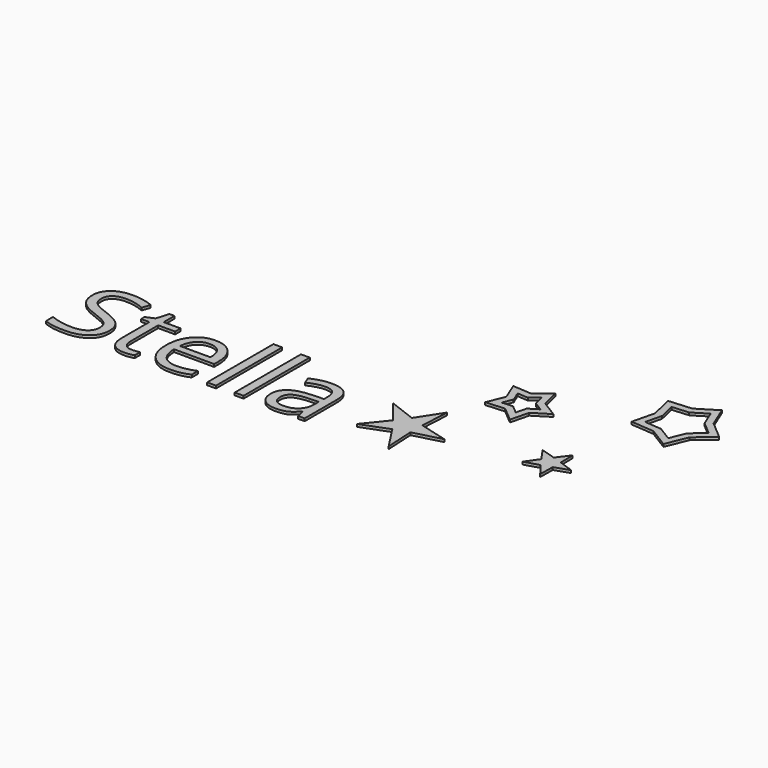
from build123d import *

# Parameters (mm, degrees)
F0_TEXT_SIZE = 12.7545618733
F1_DEPTH     = 0.3


# Not quite as in the source:
# - Text() gives the source's letters only with a copy of the font that has no kerning and outlines rounded to 1/6400 em; it was checked with that copy


with BuildPart() as f1:
    # F0 (on Top) → F1 (new body)
    with BuildSketch(Plane.XY):
        Polygon((45.5197678753, 19.2148680571), (42.8062423837, 19.0067321436), (43.4468188584, 16.3616985083), (42.8062423837, 13.7166648729), (45.5197678753, 13.5085289594), (47.8373953331, 12.0819441849), (48.8738698415, 14.5983427514), (50.9468188584, 16.3616985083), (48.8738698415, 18.1250542651), (47.8373953331, 20.6414528316), align=None)
        Polygon((47.4558552841, 19.467193304), (48.2079466306, 17.641232732), (49.7121293236, 16.3616985083), (48.2079466306, 15.0821642845), (47.4558552841, 13.2562037126), (45.7741279079, 14.2913686445), (43.8051272001, 14.4423971726), (44.2699452149, 16.3616985083), (43.8051272001, 18.2809998439), (45.7741279079, 18.4320283721), align=None, mode=Mode.SUBTRACT)
        Polygon((32.15595247, 12.3196945685), (29.9424269785, 12.4748299189), (30.7739864588, 10.4175815359), (29.9424269785, 8.3603331529), (32.15595247, 8.5154685033), (33.8555459391, 7.0888837288), (34.3920204475, 9.2420110313), (36.2739864588, 10.4175815359), (34.3920204475, 11.5931520405), (33.8555459391, 13.7462793429), align=None)
        Polygon((33.3889164299, 12.3101413844), (33.6939336388, 11.0859622857), (34.7639416466, 10.4175815359), (33.6939336388, 9.7492007861), (33.3889164299, 8.5250216874), (32.4225979039, 9.3361187653), (31.1640788938, 9.2479152238), (31.6368692086, 10.4175815359), (31.1640788938, 11.587247848), (32.4225979039, 11.4990443064), align=None, mode=Mode.SUBTRACT)
        Polygon((41.6785921238, 3.7183704865), (39.9650666323, 4.236777101), (40.9876091182, 2.7673139703), (39.9650666323, 1.2978508395), (41.6785921238, 1.816257454), (42.7601516042, 0.3896726795), (42.7966261126, 2.179528718), (44.4876091182, 2.7673139703), (42.7966261126, 3.3550992225), (42.7601516042, 5.144955261), align=None)
        Polygon((26.6473156337, 1.7384390408), (23.4702646506, 2.9568879016), (25.6108411252, 0.3118542663), (23.4702646506, -2.333179369), (26.6473156337, -1.1147305081), (28.5014175999, -3.967900057), (28.3243666168, -0.5698236121), (31.6108411252, 0.3118542663), (28.3243666168, 1.1935321448), (28.5014175999, 4.5916085897), align=None)
        with Locations((-12.1212715749, -4.444239849)):
            Text('Stella', F0_TEXT_SIZE, font='Open Sans', text_align=(TextAlign.LEFT, TextAlign.BOTTOM))
    extrude(amount=F1_DEPTH)


solid = f1.part
